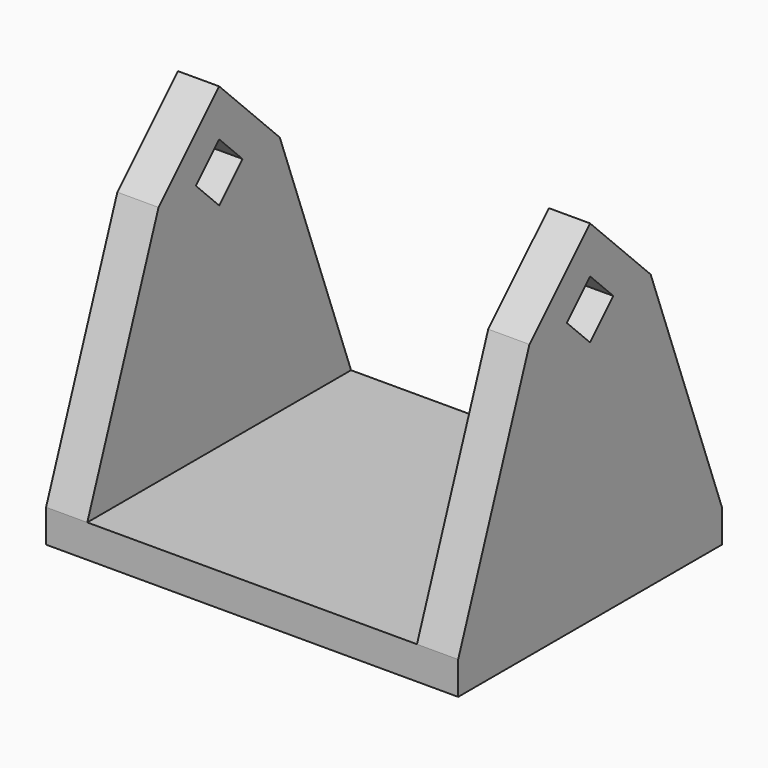
from build123d import *

# Parameters (mm, degrees)
F2_DEPTH = 2.5
F3_W     = 25
F3_H     = 20
F4_DEPTH = 2


# Not quite as in the source:
# - a pattern or mirror of a feature is missing from the dataset's text; its kind, count and spacing are read off the source's solid


with BuildPart() as f2:
    # F1 (on offset) → F2 (new body)
    with BuildSketch(Plane.YZ.offset(10)):
        Polygon((-4.5961940777, 14.6293006837), (-10, 0), (10, 0), (4.5961940777, 14.6293006837), (0, 19.2254947614), align=None)
        Polygon((0, 16.3970676367), (1.767766953, 14.6293006837), (0, 12.8615337308), (-1.767766953, 14.6293006837), align=None, mode=Mode.SUBTRACT)
    extrude(amount=F2_DEPTH)


with BuildPart() as f2_copies_1:
    # F2_copies: instance of F2
    add(f2.part.mirror(Plane(origin=(0, 0, 0), x_dir=(0, 0, -1), z_dir=(-1, 0, 0))))


with BuildPart() as f2_1:
    add(f2.part)

    add(f2_copies_1.part)  # F4 merges F2_copies_1
    # F3 (on Top) → F4 (join)
    with BuildSketch(Plane.XY):
        Rectangle(F3_W, F3_H)
    extrude(amount=-F4_DEPTH)


solid = f2_1.part
